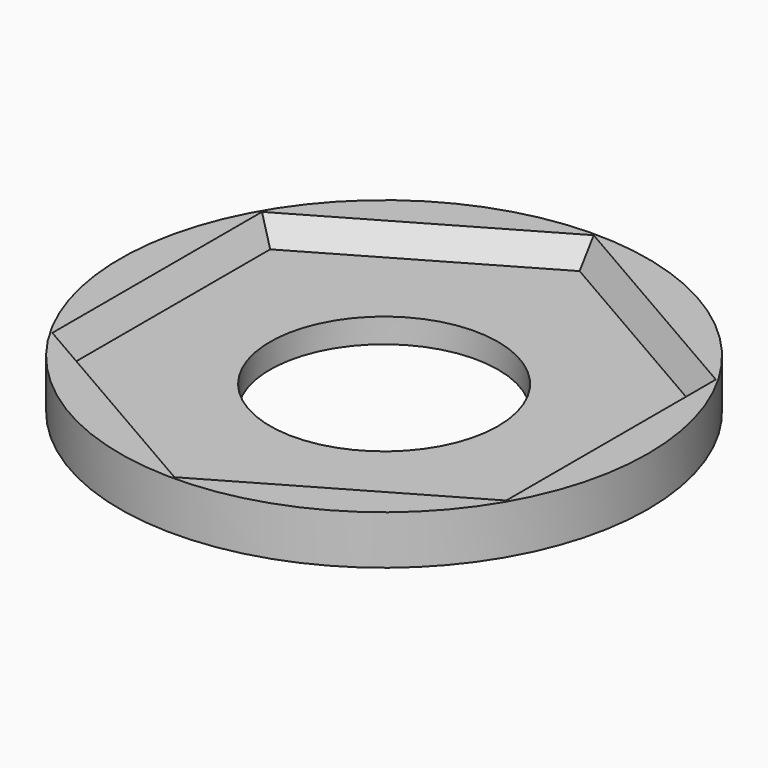
from build123d import *

# Parameters (mm, degrees)
F0_R                   = 32.4
F1_DEPTH               = 6
F0_R_2                 = 14
F2_DEPTH               = 3
F3_DEPTH               = 25
DRAFT_F3_DRAFTED_ANGLE = -32


# Not quite as in the source:
# - an extrude with a draft is written as a straight extrude whose walls are then drafted


with BuildPart() as f1:
    # F0 (on Top) → F1 (new body)
    with BuildSketch(Plane.XY):
        Circle(F0_R)
        with BuildLine():
            ThreePointArc((25.9807621135, 15), (28.9777747887, 7.7645713531), (30, 0))
            ThreePointArc((30, 0), (28.9777747887, -7.7645713531), (25.9807621135, -15))
            ThreePointArc((25.9807621135, -15), (15, -25.9807621135), (0, -30))
            ThreePointArc((0, -30), (-15, -25.9807621135), (-25.9807621135, -15))
            ThreePointArc((-25.9807621135, -15), (-30, 0), (-25.9807621135, 15))
            ThreePointArc((-25.9807621135, 15), (-15, 25.9807621135), (0, 30))
            ThreePointArc((0, 30), (15, 25.9807621135), (25.9807621135, 15))
        make_face(mode=Mode.SUBTRACT)
        with BuildLine():
            ThreePointArc((0, -30), (15, -25.9807621135), (25.9807621135, -15))
            Line((25.9807621135, -15), (0, -30))
        make_face()
        with BuildLine():
            ThreePointArc((25.9807621135, -15), (28.9777747887, -7.7645713531), (30, 0))
            ThreePointArc((30, 0), (28.9777747887, 7.7645713531), (25.9807621135, 15))
            Line((25.9807621135, 15), (25.9807621135, -15))
        make_face()
        with BuildLine():
            Line((0, 30), (25.9807621135, 15))
            ThreePointArc((25.9807621135, 15), (15, 25.9807621135), (0, 30))
        make_face()
        with BuildLine():
            Line((-25.9807621135, 15), (0, 30))
            ThreePointArc((0, 30), (-15, 25.9807621135), (-25.9807621135, 15))
        make_face()
        with BuildLine():
            Line((-25.9807621135, -15), (-25.9807621135, 15))
            ThreePointArc((-25.9807621135, 15), (-30, 0), (-25.9807621135, -15))
        make_face()
        with BuildLine():
            ThreePointArc((-25.9807621135, -15), (-15, -25.9807621135), (0, -30))
            Line((0, -30), (-25.9807621135, -15))
        make_face()
    extrude(amount=F1_DEPTH)

    # F0 (on Top) → F2 (join)
    with BuildSketch(Plane.XY):
        Polygon((25.9807621135, -15), (25.9807621135, 15), (0, 30), (-25.9807621135, 15), (-25.9807621135, -15), (0, -30), align=None)
        Circle(F0_R_2, mode=Mode.SUBTRACT)
    extrude(amount=F2_DEPTH)


with BuildPart() as f3_drafted:
    # F3 (new): a face of the model
    f3_faces = [f1.part.faces().sort_by_distance(p)[0] for p in [
        (25.1870367202, 0, 3),
    ]]
    extrude(f3_faces, amount=F3_DEPTH)

    # draft_F3_drafted
    draft_f3_drafted_walls = [f3_drafted.faces().sort_by_distance(p)[0] for p in [
        (25.9807621135, 0, 19.6666666667),
        (12.9903810568, 22.5, 19.6666666667),
        (-12.9903810568, 22.5, 19.6666666667),
        (-25.9807621135, 0, 19.6666666667),
        (-12.9903810568, -22.5, 19.6666666667),
        (12.9903810568, -22.5, 19.6666666667),
        (-14, 0, 19.6666666667),
    ]]
    draft(draft_f3_drafted_walls, neutral_plane=Plane.XY.offset(3), angle=DRAFT_F3_DRAFTED_ANGLE)


with BuildPart() as f1_1:
    add(f1.part)

    # join_F3_drafted: cut F3_drafted
    add(f3_drafted.part, mode=Mode.SUBTRACT)


solid = f1_1.part
